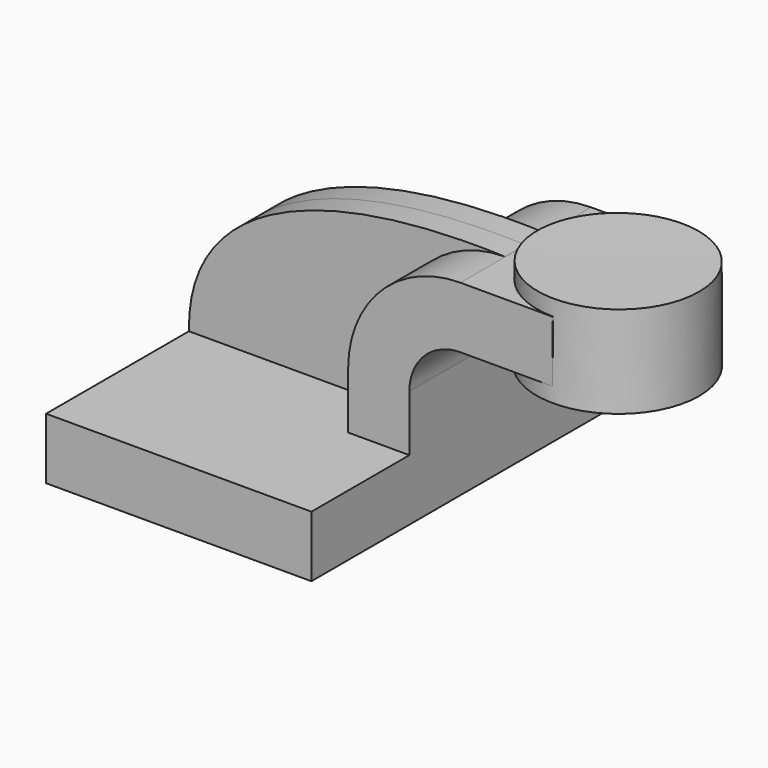
from build123d import *

# Parameters (mm, degrees)
F1_DEPTH    = 63.5
F2_DEPTH    = 25.4
F3_DEPTH    = 7.9375
F5_T1_DEPTH = 7.9375
F5_T3_DEPTH = 7.9375
F5_T8_DEPTH = 8.0594365629


# Not quite as in the source:
# - a fillet or chamfer that OpenCascade refuses, or shapes differently, is made with other operations: its cross-section is extruded or revolved along the edge and cut away or added


with BuildPart() as f1:
    # F0 (on Front) → F1 (new body, symmetric)
    with BuildSketch(Plane.XZ):
        Polygon((-41.275, 9.525), (-41.275, -9.525), (41.275, -9.525), (41.275, 9.525), (22.2249999642, 9.525), align=None)
    extrude(amount=F1_DEPTH, both=True)

    # F0 (on Front) → F2 (join, symmetric)
    with BuildSketch(Plane.XZ):
        with BuildLine():
            Line((22.2249999642, 9.525), (41.275, 9.525))
            Line((41.275, 9.525), (41.275, 27.0002))
            ThreePointArc((41.275, 27.0002), (45.9246798487, 38.2255201513), (57.15, 42.8752))
            Line((57.15, 42.8752), (60.325, 42.8752))
            Line((60.325, 42.8752), (60.325, 61.9252000358))
            Line((60.325, 61.9252000358), (57.15, 61.9252000358))
            ThreePointArc((57.15, 61.9252000358), (32.4542956418, 51.6959043582), (22.2249999642, 27.0002))
            Line((22.2249999642, 27.0002), (22.2249999642, 9.525))
        make_face()
        Polygon((85.8965185289, 61.9252000358), (60.325, 61.9252000358), (60.325, 42.8752), (85.759376848, 42.8752), align=None)
    extrude(amount=F2_DEPTH, both=True)

    # F0 (on Front) → F3 (join, symmetric)
    with BuildSketch(Plane.XZ):
        with BuildLine():
            add(Edge.make_bspline(
                [(-41.275, 9.525), (-42.0210659504, 47.4507585168), (0, 63.975892961), (57.15, 61.9252000358)],
                knots=[0, 0, 0, 0, 111.5045361803, 111.5045361803, 111.5045361803, 111.5045361803], degree=3))
            Line((-41.275, 9.525), (22.2249999642, 9.525))
            Line((22.2249999642, 9.525), (22.2249999642, 27.0002))
            ThreePointArc((22.2249999642, 27.0002), (32.4542956418, 51.6959043582), (57.15, 61.9252000358))
        make_face()
    extrude(amount=F3_DEPTH, both=True)

    # F0 (on Front) → F4 (revolve)
    with BuildSketch(Plane.XZ):
        Polygon((85.9307125211, 66.675), (85.8965185289, 61.9252000358), (85.759376848, 42.8752), (85.725, 38.1), (111.125, 38.1), (111.125, 66.675), align=None)
    revolve(axis=Axis((85.8278562605, 0, 52.3875), (0.0071988518, 0, 0.9999740879)))

    # F5: fillet of radius 5.08 on 6 edges, made by hand

    # F5_s2 → F5_t1 (join)
    with BuildSketch(Plane.XZ):
        with BuildLine():
            ThreePointArc((57.0602012116, 61.9284074084), (57.1504319335, 61.9260019422), (57.2406911513, 61.9252000358))
            Line((57.2406911513, 61.9252000358), (57.2406911513, 61.8236000358))
            Line((57.2406911513, 61.8236000358), (57.15, 61.8236000358))
            Line((57.15, 61.8236000358), (57.1463566684, 61.8236653809))
            ThreePointArc((57.1463566684, 61.8236653809), (57.1014741691, 61.8252721742), (57.0565914128, 61.8268715558))
            Line((57.0565914128, 61.8268715558), (57.0602012116, 61.9284074084))
        make_face()
    extrude(amount=F5_T1_DEPTH)

    # F5_s4 → F5_t3 (join)
    with BuildSketch(Plane.XZ.offset(-7.9375)):
        with BuildLine():
            ThreePointArc((57.0602012116, 61.9284074084), (57.1504319335, 61.9260019422), (57.2406911513, 61.9252000358))
            Line((57.2406911513, 61.9252000358), (57.2406911513, 61.8236000358))
            Line((57.2406911513, 61.8236000358), (57.15, 61.8236000358))
            Line((57.15, 61.8236000358), (57.1463566684, 61.8236653809))
            ThreePointArc((57.1463566684, 61.8236653809), (57.1014741691, 61.8252721742), (57.0565914128, 61.8268715558))
            Line((57.0565914128, 61.8268715558), (57.0602012116, 61.9284074084))
        make_face()
    extrude(amount=F5_T3_DEPTH)


with BuildPart() as f5_tool6:
    # F5_s7 → F5_t8 (new body)
    with BuildSketch(Plane.XZ.offset(0.1219365629)):
        with BuildLine():
            ThreePointArc((-41.275, 9.4762253748), (-41.2752233916, 9.5238657859), (-41.2758935468, 9.5715020071))
            Line((-41.2758935468, 9.5715020071), (-41.1743114177, 9.5734075397))
            ThreePointArc((-41.1743114177, 9.5734075397), (-41.1738708312, 9.5502028132), (-41.1734196528, 9.526998263))
            Line((-41.1734196528, 9.526998263), (-41.1734, 9.525))
            Line((-41.1734, 9.525), (-41.1734, 9.4762253748))
            Line((-41.1734, 9.4762253748), (-41.275, 9.4762253748))
        make_face()
    extrude(amount=-F5_T8_DEPTH)

    split(bisect_by=Plane.XY.offset(9.525), keep=Keep.BOTTOM)


with BuildPart() as f1_1:
    add(f1.part)

    # F5_t5: union F5_tool6
    add(f5_tool6.part)


solid = f1_1.part
